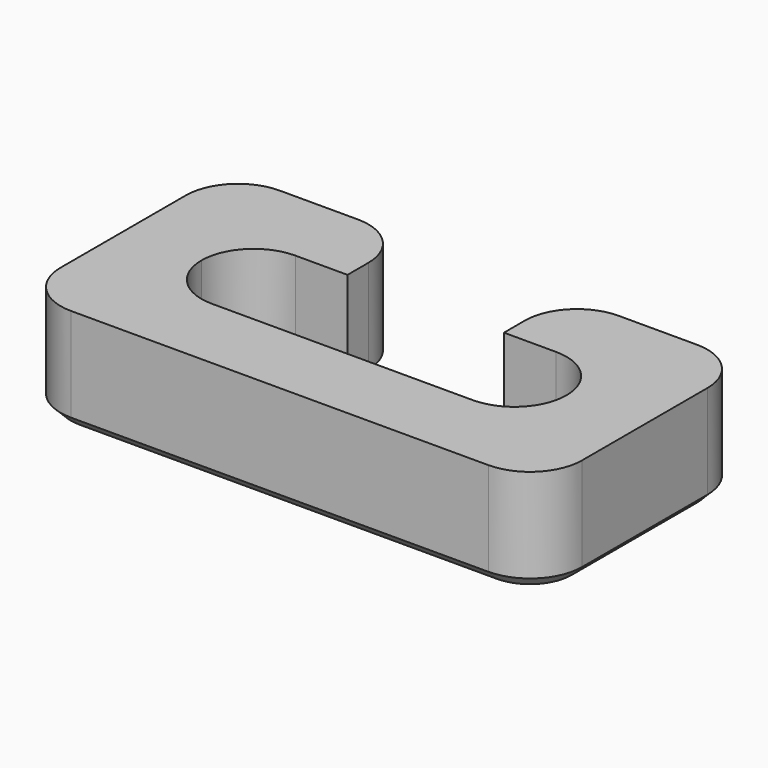
from build123d import *

# Parameters (mm, degrees)
F1_DEPTH = 2
F2_R     = 0.99999
F3_SIZE  = 0.2


# Not quite as in the source:
# - a fillet or chamfer is up to 0.001 mm smaller than in the source, because OpenCascade refuses the exact size


with BuildPart() as f1:
    # F0 (on Top) → F1 (new body)
    with BuildSketch(Plane.XY):
        Polygon((3.5, 0), (0, 0), (-3.5, 0), (-3.5, 2), (-1.5, 2), (-1.5, 3.5), (-5, 3.5), (-5, -1.5), (0, -1.5), (5, -1.5), (5, 3.5), (1.5, 3.5), (1.5, 2), (3.5, 2), align=None)
    extrude(amount=F1_DEPTH)

    # F2 (radius 1 in the source; OpenCascade refuses exactly that, so slightly less here)
    f2_edges = [f1.edges().sort_by_distance(p)[0] for p in [
        (-1.5, 3.5, 1),
        (1.5, 3.5, 1),
        (5, 3.5, 1),
        (5, -1.5, 1),
        (-5, -1.5, 1),
        (-5, 3.5, 1),
        (-3.5, 2, 1),
        (-3.5, 0, 1),
        (3.5, 2, 1),
        (3.5, 0, 1),
    ]]
    fillet(f2_edges, radius=F2_R)

    # F3
    f3_edges = [f1.edges().sort_by_distance(p)[0] for p in [
        (0, 0, 0),
        (3.20711, 0.29289, 0),
        (-3.20711, 0.29289, 0),
        (3.5, 1, 0),
        (-3.5, 1, 0),
        (3.20711, 1.70711, 0),
        (-3.20711, 1.70711, 0),
        (2.000005, 2, 0),
        (-2.000005, 2, 0),
        (1.5, 2.250005, 0),
        (-1.5, 2.250005, 0),
        (1.79289, 3.20711, 0),
        (-1.79289, 3.20711, 0),
        (3.25, 3.5, 0),
        (-3.25, 3.5, 0),
        (4.70711, 3.20711, 0),
        (-4.70711, 3.20711, 0),
        (5, 1, 0),
        (-5, 1, 0),
        (4.70711, -1.20711, 0),
        (-4.70711, -1.20711, 0),
        (0, -1.5, 0),
    ]]
    chamfer(f3_edges, length=F3_SIZE)


solid = f1.part
